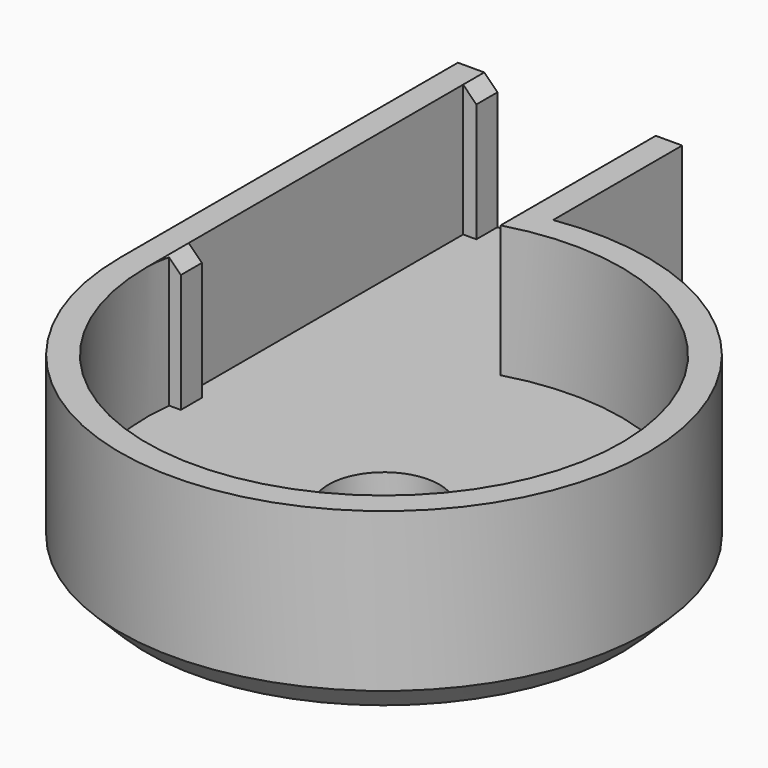
from build123d import *

# Parameters (mm, degrees)
F0_R      = 10
F0_R_2    = 2.1
F1_DEPTH  = 7
F2_R      = 9
F3_DEPTH  = 5
F5_DEPTH  = 7
F6_W      = 8.5
F6_H      = 2
F7_DEPTH  = 12.8
F8_W      = 6.5
F8_H      = 5
F9_DEPTH  = 15
F10_W     = 1
F10_H     = 5
F11_DEPTH = 0.5
F12_W     = 1
F12_H     = 5
F13_DEPTH = 0.5
F14_SIZE  = 0.49999
F15_SIZE  = 1


# Not quite as in the source:
# - a fillet or chamfer is up to 0.001 mm smaller than in the source, because OpenCascade refuses the exact size


with BuildPart() as f1:
    # F0 (on Top) → F1 (new body)
    with BuildSketch(Plane.XY):
        Circle(F0_R)
        Circle(F0_R_2, mode=Mode.SUBTRACT)
    extrude(amount=F1_DEPTH)

    # F2 (on face) → F3 (cut)
    with BuildSketch(Plane.XY.offset(7)):
        Circle(F2_R)
    extrude(amount=-F3_DEPTH, mode=Mode.SUBTRACT)

    # F4 (on face) → F5 (join)
    with BuildSketch(Plane.XY.offset(7)):
        with BuildLine():
            Line((-10, 16), (-10, 0))
            ThreePointArc((-10, 0), (-9.7467943448, 2.2360679775), (-9, 4.3588989435))
            Line((-9, 4.3588989435), (-9, 16))
            Line((-9, 16), (-10, 16))
        make_face()
        with BuildLine():
            ThreePointArc((-2.5, 9.6824583655), (-2.0026095485, 9.7974259373), (-1.5, 9.8868599666))
            Line((-1.5, 9.8868599666), (-1.5, 16))
            Line((-1.5, 16), (-2.5, 16))
            Line((-2.5, 16), (-2.5, 9.6824583655))
        make_face()
    extrude(amount=-F5_DEPTH)

    # F6 (on face) → F7 (join)
    with BuildSketch(Plane(origin=(0, 16, 0), x_dir=(-1, 0, 0), z_dir=(0, 1, 0))):
        with Locations((5.75, 1)):
            Rectangle(F6_W, F6_H)
    extrude(amount=-F7_DEPTH)

    # F8 (on face) → F9 (cut)
    with BuildSketch(Plane(origin=(0, 16, 0), x_dir=(-1, 0, 0), z_dir=(0, 1, 0))):
        with Locations((5.75, 4.5)):
            Rectangle(F8_W, F8_H)
    extrude(amount=-F9_DEPTH, mode=Mode.SUBTRACT)

    # F10 (on face) → F11 (join)
    with BuildSketch(Plane.YZ.offset(-9)):
        with Locations((1.5, 4.5)):
            Rectangle(F10_W, F10_H)
        with Locations((15.5, 4.5)):
            Rectangle(F10_W, F10_H)
    extrude(amount=F11_DEPTH)

    # F12 (on face) → F13 (join)
    with BuildSketch(Plane(origin=(-2.5, 0, 0), x_dir=(0, -1, 0), z_dir=(-1, 0, 0))):
        with Locations((-15.5, 4.5)):
            Rectangle(F12_W, F12_H)
    extrude(amount=F13_DEPTH)

    # F14 (size 0.5 in the source; OpenCascade refuses exactly that, so slightly less here)
    f14_edges = [f1.edges().sort_by_distance(p)[0] for p in [
        (-8.5, 1.5, 7),
        (-8.5, 15.5, 7),
        (-3, 15.5, 7),
    ]]
    chamfer(f14_edges, length=F14_SIZE)

    # F15
    f15_edges = [f1.edges().sort_by_distance(p)[0] for p in [
        (7.582875, -6.519202, 0),
        (-1.5, 12.94343, 0),
        (-10, 8, 0),
    ]]
    chamfer(f15_edges, length=F15_SIZE)


solid = f1.part
